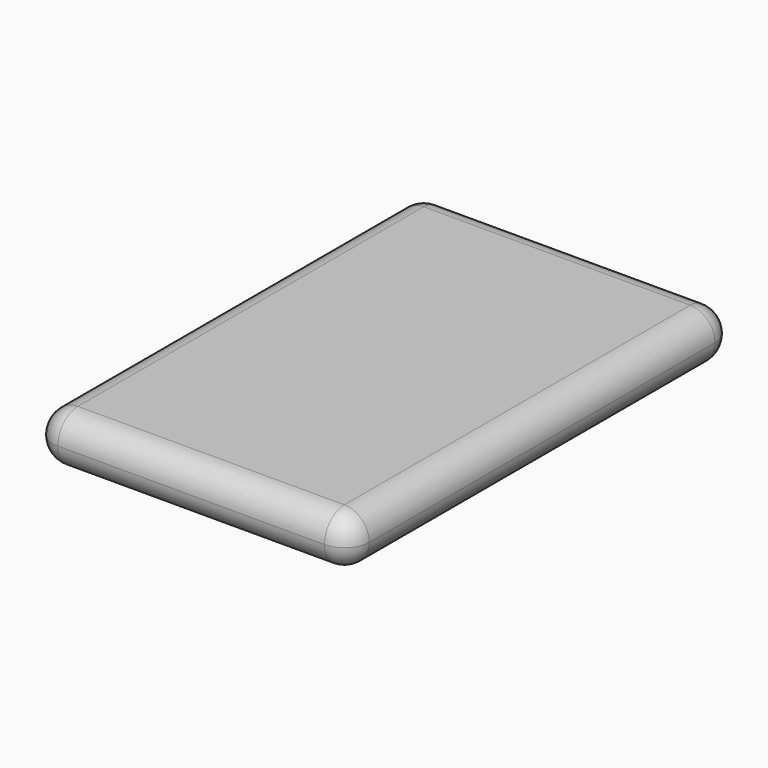
from build123d import *

# Parameters (mm, degrees)
F0_W     = 63.6741071939
F0_H     = 97.0434620976
F1_DEPTH = 10
F2_R     = 4.99999


# Not quite as in the source:
# - a fillet or chamfer is up to 0.001 mm smaller than in the source, because OpenCascade refuses the exact size


with BuildPart() as f1:
    # F0 (on Top) → F1 (new body)
    with BuildSketch(Plane.XY):
        with Locations((-11.2950801849, -8.3157271147)):
            Rectangle(F0_W, F0_H)
    extrude(amount=F1_DEPTH)

    # F2 (radius 5 in the source; OpenCascade refuses exactly that, so slightly less here)
    f2_edges = [f1.edges().sort_by_distance(p)[0] for p in [
        (20.541973, -56.837458, 5),
        (20.541973, 40.206004, 5),
        (20.541973, -8.315727, 0),
        (20.541973, -8.315727, 10),
        (-43.132134, 40.206004, 5),
        (-11.29508, 40.206004, 0),
        (-11.29508, 40.206004, 10),
        (-43.132134, -56.837458, 5),
        (-43.132134, -8.315727, 0),
        (-43.132134, -8.315727, 10),
        (-11.29508, -56.837458, 0),
        (-11.29508, -56.837458, 10),
    ]]
    fillet(f2_edges, radius=F2_R)


solid = f1.part
